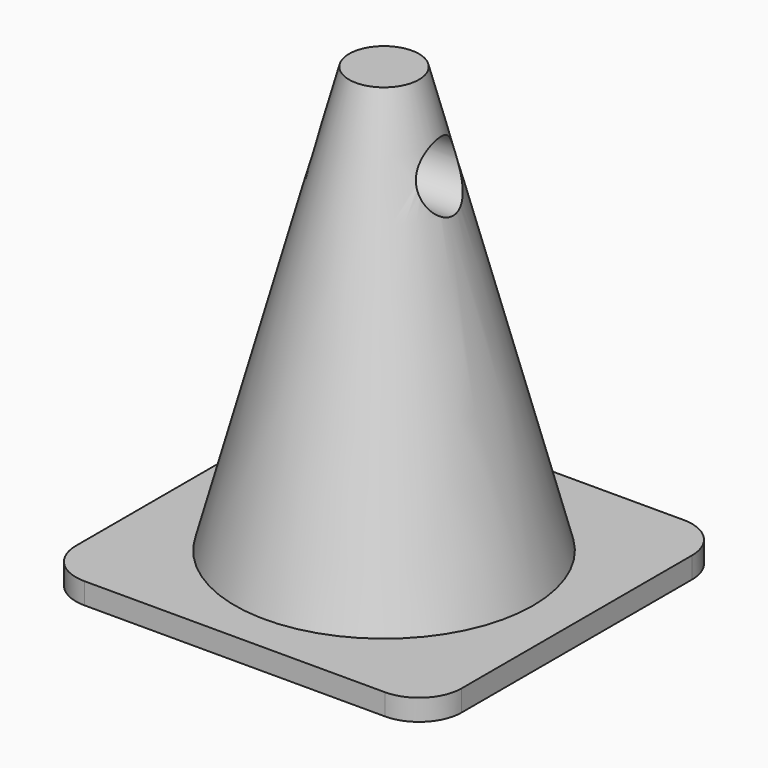
from build123d import *

# Parameters (mm, degrees)
F0_R     = 17.5
F1_DEPTH = 2.5
F2_R     = 17.5
F3_DEPTH = 50
F3_TAPER = 15
F4_R     = 3.6137849114
F5_DEPTH = 60


with BuildPart() as f1:
    # F0 (on Top) → F1 (new body)
    with BuildSketch(Plane.XY):
        with BuildLine():
            Line((0, 38.8068709316), (-35.2930977718, 38.8068709316))
            ThreePointArc((-35.2930977718, 38.8068709316), (-38.8286316778, 37.3424048375), (-40.2930977718, 33.8068709316))
            Line((-40.2930977718, 33.8068709316), (-40.2930977718, 0))
            ThreePointArc((-40.2930977718, 0), (-38.8286316778, -3.5355339059), (-35.2930977718, -5))
            Line((-35.2930977718, -5), (0, -5))
            ThreePointArc((0, -5), (3.5355339059, -3.5355339059), (5, 0))
            Line((5, 0), (5, 33.8068709316))
            ThreePointArc((5, 33.8068709316), (3.5355339059, 37.3424048375), (0, 38.8068709316))
        make_face()
        with Locations((-17.6465488859, 16.9034354658)):
            Circle(F0_R, mode=Mode.SUBTRACT)
        with Locations((-17.6465488859, 16.9034354658)):
            Circle(F0_R)
    extrude(amount=F1_DEPTH)

    # F2 (on face) → F3 (join)
    with BuildSketch(Plane.XY.offset(2.5)):
        with Locations((-17.6465488859, 16.9034354658)):
            Circle(F2_R)
    extrude(amount=F3_DEPTH, taper=F3_TAPER)

    # F4 (on Right) → F5 (cut)
    with BuildSketch(Plane.YZ):
        with Locations((17.7631601691, 42.927633971)):
            Circle(F4_R)
    extrude(amount=-F5_DEPTH, mode=Mode.SUBTRACT)


solid = f1.part
